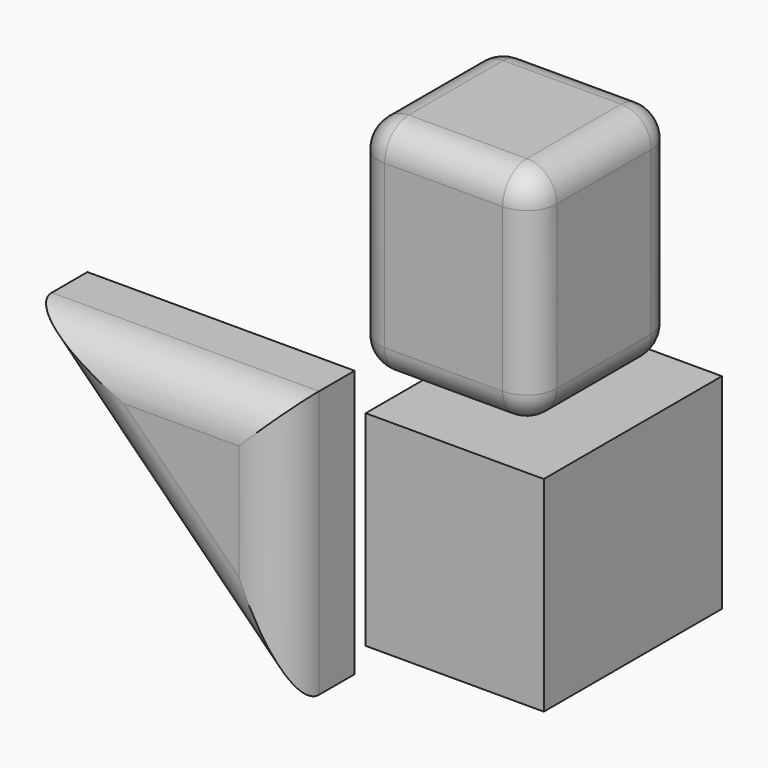
from build123d import *

# Parameters (mm, degrees)
F0_W         = 50.8
F0_H         = 50.8
F1_DEPTH     = 63.5
F2_R         = 15.8771693286
F3_DEPTH     = 25.4
F5_T3_DEPTH  = 46.3301131444
F5_T5_DEPTH  = 33.6301131444
F5_T7_DEPTH  = 33.6301131444
F5_S11_W     = 8.5849434278
F5_S11_H     = 8.5849434278
F5_T12_DEPTH = 8.5849434278
F5_S17_W     = 8.5849434278
F5_S17_H     = 8.5849434278
F5_T18_DEPTH = 8.5849434278
F5_S23_W     = 8.5849434278
F5_S23_H     = 8.5849434278
F5_T24_DEPTH = 8.5849434278
F5_S29_W     = 8.5849434278
F5_S29_H     = 8.5849434278
F5_T30_DEPTH = 8.5849434278
F5_S35_W     = 8.5849434278
F5_S35_H     = 8.5849434278
F5_T36_DEPTH = 8.5849434278
F5_S41_W     = 8.5849434278
F5_S41_H     = 8.5849434278
F5_T42_DEPTH = 8.5849434278
F5_S47_W     = 8.5849434278
F5_S47_H     = 8.5849434278
F5_T48_DEPTH = 8.5849434278
F5_S53_W     = 8.5849434278
F5_S53_H     = 8.5849434278
F5_T54_DEPTH = 8.5849434278
F7_DEPTH     = 25.4
F8_R         = 12.7
F9_W         = 63.5
F9_H         = 58.42
F10_DEPTH    = 50.8


# Not quite as in the source:
# - a fillet or chamfer that OpenCascade refuses, or shapes differently, is made with other operations: its cross-section is extruded or revolved along the edge and cut away or added


with BuildPart() as f1:
    # F0 (on Top) → F1 (new body)
    with BuildSketch(Plane.XY):
        with Locations((25.4, 25.4)):
            Rectangle(F0_W, F0_H)
    extrude(amount=F1_DEPTH)


with BuildPart() as f3:
    # F2 (on Top) → F3 (new body)
    with BuildSketch(Plane.XY):
        with Locations((23.6034151167, 27.0417090505)):
            Circle(F2_R)
    extrude(amount=F3_DEPTH)


with BuildPart() as f1_1:
    add(f1.part)

    # F4: cut F3
    add(f3.part, mode=Mode.SUBTRACT)

    # F5: fillet of radius 8.5849434278 on 14 edges, made by hand

    # F5_s1 → F5_t2 (revolve)
    with BuildSketch(Plane.XZ.offset(-27.0417090505)):
        with BuildLine():
            ThreePointArc((39.4805844452, 16.8150565722), (36.9661127313, 22.8855282861), (30.8956410174, 25.4))
            Line((30.8956410174, 25.4), (39.4805844452, 25.4))
            Line((39.4805844452, 25.4), (39.4805844452, 16.8150565722))
        make_face()
    revolve(axis=Axis((23.6034151167, 27.0417090505, 25.4), (0, 0, 1)))

    # F5_s4 → F5_t3 (cut)
    with BuildSketch(Plane.XY.offset(8.5849434278)):
        with BuildLine():
            ThreePointArc((0, 42.2150565722), (2.5144717139, 48.2855282861), (8.5849434278, 50.8))
            Line((8.5849434278, 50.8), (0, 50.8))
            Line((0, 50.8), (0, 42.2150565722))
        make_face()
        with BuildLine():
            ThreePointArc((0, 8.5849434278), (2.5144717139, 2.5144717139), (8.5849434278, 0))
            Line((8.5849434278, 0), (0, 0))
            Line((0, 0), (0, 8.5849434278))
        make_face()
        with BuildLine():
            ThreePointArc((42.2150565722, 50.8), (48.2855282861, 48.2855282861), (50.8, 42.2150565722))
            Line((50.8, 42.2150565722), (50.8, 50.8))
            Line((50.8, 50.8), (42.2150565722, 50.8))
        make_face()
        with BuildLine():
            ThreePointArc((42.2150565722, 0), (48.2855282861, 2.5144717139), (50.8, 8.5849434278))
            Line((50.8, 8.5849434278), (50.8, 0))
            Line((50.8, 0), (42.2150565722, 0))
        make_face()
    extrude(amount=F5_T3_DEPTH, mode=Mode.SUBTRACT)

    # F5_s6 → F5_t5 (cut)
    with BuildSketch(Plane.XZ.offset(-42.2150565722)):
        with BuildLine():
            ThreePointArc((0, 8.5849434278), (2.5144717139, 2.5144717139), (8.5849434278, 0))
            Line((8.5849434278, 0), (0, 0))
            Line((0, 0), (0, 8.5849434278))
        make_face()
        with BuildLine():
            ThreePointArc((0, 54.9150565722), (2.5144717139, 60.9855282861), (8.5849434278, 63.5))
            Line((8.5849434278, 63.5), (0, 63.5))
            Line((0, 63.5), (0, 54.9150565722))
        make_face()
        with BuildLine():
            ThreePointArc((42.2150565722, 0), (48.2855282861, 2.5144717139), (50.8, 8.5849434278))
            Line((50.8, 8.5849434278), (50.8, 0))
            Line((50.8, 0), (42.2150565722, 0))
        make_face()
        with BuildLine():
            ThreePointArc((42.2150565722, 63.5), (48.2855282861, 60.9855282861), (50.8, 54.9150565722))
            Line((50.8, 54.9150565722), (50.8, 63.5))
            Line((50.8, 63.5), (42.2150565722, 63.5))
        make_face()
    extrude(amount=F5_T5_DEPTH, mode=Mode.SUBTRACT)

    # F5_s8 → F5_t7 (cut)
    with BuildSketch(Plane.YZ.offset(8.5849434278)):
        with BuildLine():
            ThreePointArc((50.8, 8.5849434278), (48.2855282861, 2.5144717139), (42.2150565722, 0))
            Line((42.2150565722, 0), (50.8, 0))
            Line((50.8, 0), (50.8, 8.5849434278))
        make_face()
        with BuildLine():
            ThreePointArc((50.8, 54.9150565722), (48.2855282861, 60.9855282861), (42.2150565722, 63.5))
            Line((42.2150565722, 63.5), (50.8, 63.5))
            Line((50.8, 63.5), (50.8, 54.9150565722))
        make_face()
        with BuildLine():
            ThreePointArc((0, 8.5849434278), (2.5144717139, 2.5144717139), (8.5849434278, 0))
            Line((8.5849434278, 0), (0, 0))
            Line((0, 0), (0, 8.5849434278))
        make_face()
        with BuildLine():
            ThreePointArc((0, 54.9150565722), (2.5144717139, 60.9855282861), (8.5849434278, 63.5))
            Line((8.5849434278, 63.5), (0, 63.5))
            Line((0, 63.5), (0, 54.9150565722))
        make_face()
    extrude(amount=F5_T7_DEPTH, mode=Mode.SUBTRACT)


with BuildPart() as f5_tool10:
    # F5_s11 → F5_t12 (new body)
    with BuildSketch(Plane.YZ.offset(8.5849434278)):
        with Locations((46.5075282861, 4.2924717139)):
            Rectangle(F5_S11_W, F5_S11_H)
    extrude(amount=-F5_T12_DEPTH)

    # F5_s13 → F5_t14 (revolve, cut)
    with BuildSketch(Plane(origin=(8.5849434278, 42.2150565722, 8.5849434278), x_dir=(0, -0.7071067812, 0.7071067812), z_dir=(0, -0.7071067812, -0.7071067812))):
        with BuildLine():
            ThreePointArc((0, -8.5849434278), (8.5849434278, 0), (0, 8.5849434278))
            Line((0, 8.5849434278), (0, -8.5849434278))
        make_face()
    revolve(axis=Axis((8.5849434278, 42.2150565722, 8.5849434278), (-1, 0, 0)), mode=Mode.SUBTRACT)


with BuildPart() as f1_2:
    add(f1_1.part)

    # F5_t9: cut F5_tool10
    add(f5_tool10.part, mode=Mode.SUBTRACT)


with BuildPart() as f5_tool16:
    # F5_s17 → F5_t18 (new body)
    with BuildSketch(Plane.YZ.offset(8.5849434278)):
        with Locations((46.5075282861, 59.2075282861)):
            Rectangle(F5_S17_W, F5_S17_H)
    extrude(amount=-F5_T18_DEPTH)

    # F5_s19 → F5_t20 (revolve, cut)
    with BuildSketch(Plane(origin=(8.5849434278, 42.2150565722, 54.9150565722), x_dir=(0, -0.7071067812, -0.7071067812), z_dir=(0, 0.7071067812, -0.7071067812))):
        with BuildLine():
            ThreePointArc((0, -8.5849434278), (8.5849434278, 0), (0, 8.5849434278))
            Line((0, 8.5849434278), (0, -8.5849434278))
        make_face()
    revolve(axis=Axis((8.5849434278, 42.2150565722, 54.9150565722), (-1, 0, 0)), mode=Mode.SUBTRACT)


with BuildPart() as f1_3:
    add(f1_2.part)

    # F5_t15: cut F5_tool16
    add(f5_tool16.part, mode=Mode.SUBTRACT)


with BuildPart() as f5_tool22:
    # F5_s23 → F5_t24 (new body)
    with BuildSketch(Plane.YZ.offset(8.5849434278)):
        with Locations((4.2924717139, 4.2924717139)):
            Rectangle(F5_S23_W, F5_S23_H)
    extrude(amount=-F5_T24_DEPTH)

    # F5_s25 → F5_t26 (revolve, cut)
    with BuildSketch(Plane(origin=(8.5849434278, 8.5849434278, 8.5849434278), x_dir=(0, 0.7071067812, 0.7071067812), z_dir=(0, -0.7071067812, 0.7071067812))):
        with BuildLine():
            ThreePointArc((0, -8.5849434278), (8.5849434278, 0), (0, 8.5849434278))
            Line((0, 8.5849434278), (0, -8.5849434278))
        make_face()
    revolve(axis=Axis((8.5849434278, 8.5849434278, 8.5849434278), (-1, 0, 0)), mode=Mode.SUBTRACT)


with BuildPart() as f1_4:
    add(f1_3.part)

    # F5_t21: cut F5_tool22
    add(f5_tool22.part, mode=Mode.SUBTRACT)


with BuildPart() as f5_tool28:
    # F5_s29 → F5_t30 (new body)
    with BuildSketch(Plane.YZ.offset(8.5849434278)):
        with Locations((4.2924717139, 59.2075282861)):
            Rectangle(F5_S29_W, F5_S29_H)
    extrude(amount=-F5_T30_DEPTH)

    # F5_s31 → F5_t32 (revolve, cut)
    with BuildSketch(Plane(origin=(8.5849434278, 8.5849434278, 54.9150565722), x_dir=(0, 0.7071067812, -0.7071067812), z_dir=(0, 0.7071067812, 0.7071067812))):
        with BuildLine():
            ThreePointArc((0, -8.5849434278), (8.5849434278, 0), (0, 8.5849434278))
            Line((0, 8.5849434278), (0, -8.5849434278))
        make_face()
    revolve(axis=Axis((8.5849434278, 8.5849434278, 54.9150565722), (-1, 0, 0)), mode=Mode.SUBTRACT)


with BuildPart() as f1_5:
    add(f1_4.part)

    # F5_t27: cut F5_tool28
    add(f5_tool28.part, mode=Mode.SUBTRACT)


with BuildPart() as f5_tool34:
    # F5_s35 → F5_t36 (new body)
    with BuildSketch(Plane.XZ.offset(-42.2150565722)):
        with Locations((46.5075282861, 4.2924717139)):
            Rectangle(F5_S35_W, F5_S35_H)
    extrude(amount=-F5_T36_DEPTH)

    # F5_s37 → F5_t38 (revolve, cut)
    with BuildSketch(Plane(origin=(42.2150565722, 42.2150565722, 8.5849434278), x_dir=(-0.7071067812, 0, 0.7071067812), z_dir=(-0.7071067812, 0, -0.7071067812))):
        with BuildLine():
            ThreePointArc((0, -8.5849434278), (8.5849434278, 0), (0, 8.5849434278))
            Line((0, 8.5849434278), (0, -8.5849434278))
        make_face()
    revolve(axis=Axis((42.2150565722, 42.2150565722, 8.5849434278), (0, 1, 0)), mode=Mode.SUBTRACT)


with BuildPart() as f1_6:
    add(f1_5.part)

    # F5_t33: cut F5_tool34
    add(f5_tool34.part, mode=Mode.SUBTRACT)


with BuildPart() as f5_tool40:
    # F5_s41 → F5_t42 (new body)
    with BuildSketch(Plane.XZ.offset(-42.2150565722)):
        with Locations((46.5075282861, 59.2075282861)):
            Rectangle(F5_S41_W, F5_S41_H)
    extrude(amount=-F5_T42_DEPTH)

    # F5_s43 → F5_t44 (revolve, cut)
    with BuildSketch(Plane(origin=(42.2150565722, 42.2150565722, 54.9150565722), x_dir=(-0.7071067812, 0, -0.7071067812), z_dir=(0.7071067812, 0, -0.7071067812))):
        with BuildLine():
            ThreePointArc((0, -8.5849434278), (8.5849434278, 0), (0, 8.5849434278))
            Line((0, 8.5849434278), (0, -8.5849434278))
        make_face()
    revolve(axis=Axis((42.2150565722, 42.2150565722, 54.9150565722), (0, 1, 0)), mode=Mode.SUBTRACT)


with BuildPart() as f1_7:
    add(f1_6.part)

    # F5_t39: cut F5_tool40
    add(f5_tool40.part, mode=Mode.SUBTRACT)


with BuildPart() as f5_tool46:
    # F5_s47 → F5_t48 (new body)
    with BuildSketch(Plane.XZ.offset(-8.5849434278)):
        with Locations((46.5075282861, 4.2924717139)):
            Rectangle(F5_S47_W, F5_S47_H)
    extrude(amount=F5_T48_DEPTH)

    # F5_s49 → F5_t50 (revolve, cut)
    with BuildSketch(Plane(origin=(42.2150565722, 8.5849434278, 8.5849434278), x_dir=(-0.7071067812, 0, 0.7071067812), z_dir=(0.7071067812, 0, 0.7071067812))):
        with BuildLine():
            ThreePointArc((0, -8.5849434278), (8.5849434278, 0), (0, 8.5849434278))
            Line((0, 8.5849434278), (0, -8.5849434278))
        make_face()
    revolve(axis=Axis((42.2150565722, 8.5849434278, 8.5849434278), (0, -1, 0)), mode=Mode.SUBTRACT)


with BuildPart() as f1_8:
    add(f1_7.part)

    # F5_t45: cut F5_tool46
    add(f5_tool46.part, mode=Mode.SUBTRACT)


with BuildPart() as f5_tool52:
    # F5_s53 → F5_t54 (new body)
    with BuildSketch(Plane.XZ.offset(-8.5849434278)):
        with Locations((46.5075282861, 59.2075282861)):
            Rectangle(F5_S53_W, F5_S53_H)
    extrude(amount=F5_T54_DEPTH)

    # F5_s55 → F5_t56 (revolve, cut)
    with BuildSketch(Plane(origin=(42.2150565722, 8.5849434278, 54.9150565722), x_dir=(-0.7071067812, 0, -0.7071067812), z_dir=(-0.7071067812, 0, 0.7071067812))):
        with BuildLine():
            ThreePointArc((0, -8.5849434278), (8.5849434278, 0), (0, 8.5849434278))
            Line((0, 8.5849434278), (0, -8.5849434278))
        make_face()
    revolve(axis=Axis((42.2150565722, 8.5849434278, 54.9150565722), (0, -1, 0)), mode=Mode.SUBTRACT)


with BuildPart() as f1_9:
    add(f1_8.part)

    # F5_t51: cut F5_tool52
    add(f5_tool52.part, mode=Mode.SUBTRACT)

    # F5_s57 → F5_t58 (revolve, cut)
    with BuildSketch(Plane.XZ.offset(-27.0417090505)):
        with BuildLine():
            ThreePointArc((48.065527873, 0), (41.9950561591, 2.5144717139), (39.4805844452, 8.5849434278))
            Line((39.4805844452, 8.5849434278), (39.4805844452, 0))
            Line((39.4805844452, 0), (48.065527873, 0))
        make_face()
    revolve(axis=Axis((23.6034151167, 27.0417090505, 0), (0, 0, 1)), mode=Mode.SUBTRACT)


with BuildPart() as f7:
    # F6 (on Front) → F7 (new body)
    with BuildSketch(Plane.XZ):
        Polygon((0, -76.2), (0, 0), (-76.2, 0), align=None)
    extrude(amount=F7_DEPTH)

    # F8
    f8_edges = [f7.edges().sort_by_distance(p)[0] for p in [
        (0, -25.4, -38.1),
        (-38.1, -25.4, 0),
        (-38.1, -25.4, -38.1),
    ]]
    fillet(f8_edges, radius=F8_R)


with BuildPart() as f10:
    # F9 (on Right) → F10 (new body)
    with BuildSketch(Plane.YZ):
        with Locations((35.6839029118, -41.4694223068)):
            Rectangle(F9_W, F9_H)
    extrude(amount=F10_DEPTH)


solid = Compound([f1_9.part, f7.part, f10.part])
